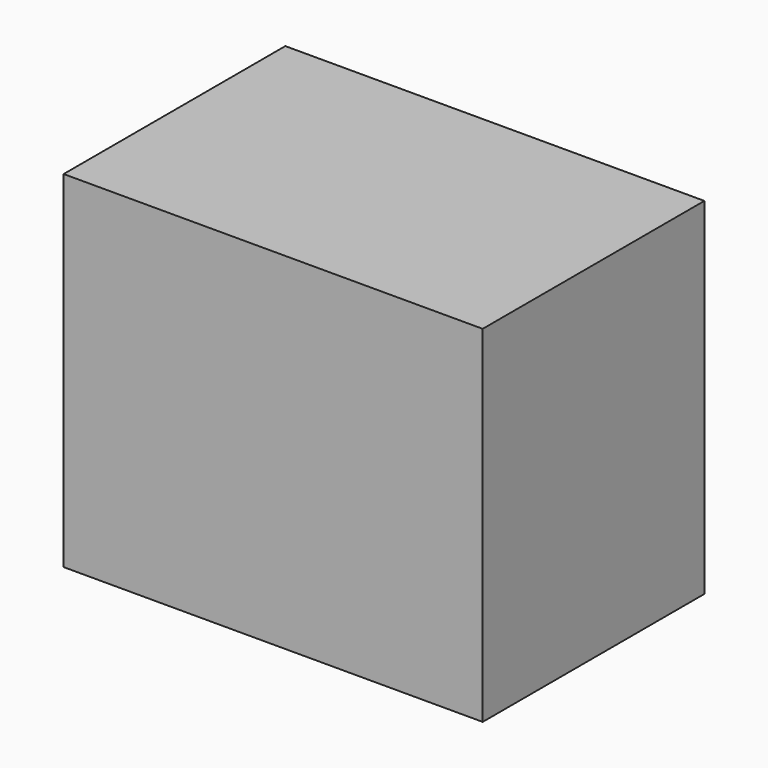
from build123d import *

# Parameters (mm, degrees)
F0_W     = 28.2447356731
F0_H     = 26.8375258893
F2_DEPTH = 25.4
F1_W     = 38.4147167206
F1_H     = 31.7230820656
F3_DEPTH = 25.4


# Not quite as in the source:
# - a feature of the source that left no trace in its solid (it failed there, or was rolled back) is left out


with BuildPart() as f2:
    # F0 (on Front) → F2 (new body)
    with BuildSketch(Plane.XZ):
        with Locations((14.1223678365, 13.4187629446)):
            Rectangle(F0_W, F0_H)
    extrude(amount=F2_DEPTH)


with BuildPart() as f3:
    # F1 (on Front) → F3 (new body)
    with BuildSketch(Plane.XZ):
        with Locations((19.2073583603, 15.8615410328)):
            Rectangle(F1_W, F1_H)
    extrude(amount=F3_DEPTH)


solid = Compound([f2.part, f3.part])
